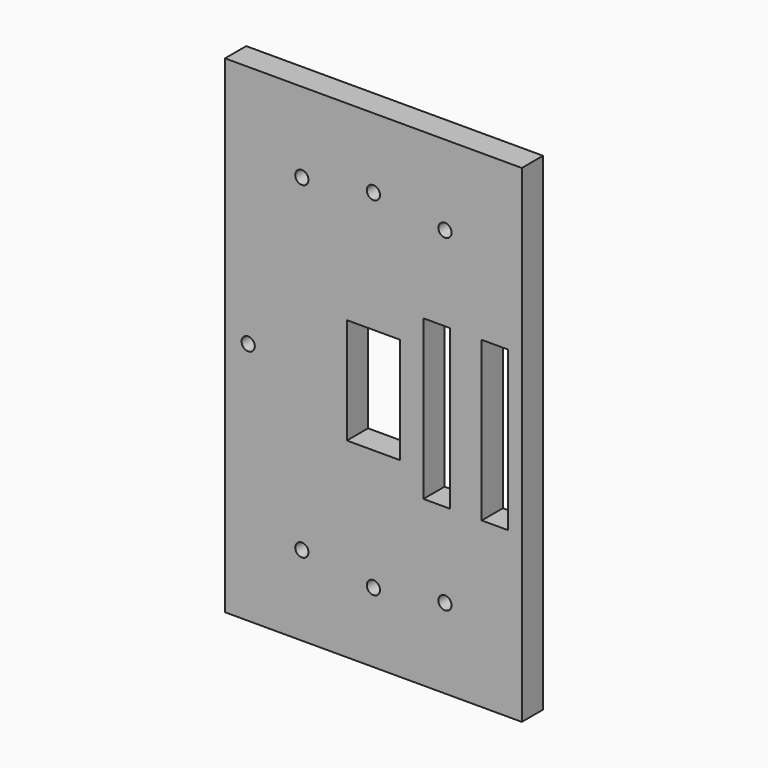
from build123d import *

# Parameters (mm, degrees)
F0_R     = 1.5875
F0_W     = 6.35
F0_H     = 38.1
F1_DEPTH = 3.175
F2_DEPTH = 2.54


# Not quite as in the source:
# - a feature names something its author has since deleted; it is built from what else it names


with BuildPart() as f1:
    # F0 (on Front) → F1 (new body, symmetric)
    with BuildSketch(Plane.XZ):
        Polygon((35.56, -58.42), (35.56, 58.42), (-35.56, 58.42), (-35.56, 0), (-35.56, -58.42), align=None)
        with Locations((-17.1425342897, -39.2875)):
            Circle(F0_R, mode=Mode.SUBTRACT)
        with Locations((0, -41.656)):
            Circle(F0_R, mode=Mode.SUBTRACT)
        with BuildLine():
            ThreePointArc((-28.4118865192, 0), (-29.9993865192, -1.5875), (-31.5868865192, 0))
            ThreePointArc((-31.5868865192, 0), (-29.9993865192, 1.5875), (-28.4118865192, 0))
        make_face(mode=Mode.SUBTRACT)
        Polygon((-6.35, -12.7), (-6.35, 12.7), (0, 12.7), (6.35, 12.7), (6.35, -12.7), align=None, mode=Mode.SUBTRACT)
        with Locations((17.1425342897, -39.2875)):
            Circle(F0_R, mode=Mode.SUBTRACT)
        with Locations((15.1556345809, 0)):
            Rectangle(F0_W, F0_H, mode=Mode.SUBTRACT)
        with Locations((29.1256345809, 0)):
            Rectangle(F0_W, F0_H, mode=Mode.SUBTRACT)
        with Locations((-17.1425342897, 39.2875)):
            Circle(F0_R, mode=Mode.SUBTRACT)
        with BuildLine():
            ThreePointArc((1.5875, 41.656), (1.1225320151, 40.5334679849), (0, 40.0685))
            ThreePointArc((0, 40.0685), (-1.1225320151, 42.7785320151), (1.5875, 41.656))
        make_face(mode=Mode.SUBTRACT)
        with Locations((17.1425342897, 39.2875)):
            Circle(F0_R, mode=Mode.SUBTRACT)
    extrude(amount=F1_DEPTH, both=True)

    # F0 (on Front) → F2 (cut)
    with BuildSketch(Plane.XZ):
        with Locations((15.1556345809, 0)):
            Rectangle(F0_W, F0_H)
        with Locations((29.1256345809, 0)):
            Rectangle(F0_W, F0_H)
    extrude(amount=-F2_DEPTH, mode=Mode.SUBTRACT)


solid = f1.part
